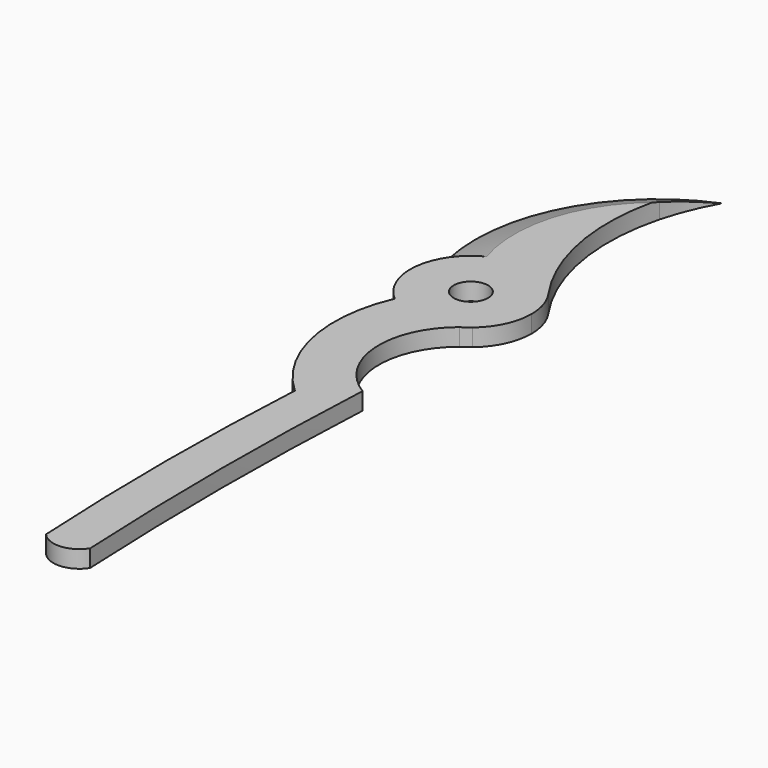
from build123d import *

# Parameters (mm, degrees)
F0_R     = 3.97
F1_DEPTH = 4
F2_SIZE2 = 3.99999
F2_SIZE  = 8.99999


# Not quite as in the source:
# - a fillet or chamfer is up to 0.001 mm smaller than in the source, because OpenCascade refuses the exact size


with BuildPart() as f1:
    # F0 (on Top) → F1 (new body)
    with BuildSketch(Plane.XY):
        with BuildLine():
            ThreePointArc((-1.9595979293, -1.3771342837), (-1.0019520075, -0.6570443939), (0, 0))
            Line((0, 0), (-18, 0))
            ThreePointArc((-18, 0), (-10.1975519696, -3.2248817144), (-1.9595979293, -1.3771342837))
        make_face()
        with BuildLine():
            Line((-18, 0), (0, 0))
            ThreePointArc((0, 0), (3.6885775404, 4.8077255117), (5, 10.7238052948))
            ThreePointArc((5, 10.7238052948), (4.3572555803, 14.9171003433), (2.4880395194, 18.7253643928))
            ThreePointArc((2.4880395194, 18.7253643928), (-5.3400778901, 24.2369459419), (-14.8797121879, 23.4292759507))
            ThreePointArc((-14.8797121879, 23.4292759507), (-19.2476875403, 20.262405825), (-22.0937623429, 15.6789428013))
            ThreePointArc((-22.0937623429, 15.6789428013), (-22.5458811252, 7.1869840464), (-18, 0))
        make_face()
        with Locations((-9, 10.7238052948)):
            Circle(F0_R, mode=Mode.SUBTRACT)
        with BuildLine():
            ThreePointArc((-1.9595979293, -1.3771342837), (-0.9502950764, -0.7305498003), (0, 0))
            ThreePointArc((0, 0), (-1.0019520075, -0.6570443939), (-1.9595979293, -1.3771342837))
        make_face()
        with BuildLine():
            ThreePointArc((-1.9595979293, -1.3771342837), (-10.1975519696, -3.2248817144), (-18, 0))
            ThreePointArc((-18, 0), (-20.1233033288, -20.9955621955), (-9.6223697705, -39.3))
            ThreePointArc((-9.6223697705, -39.3), (-10.6300458729, -75.2), (-9.6223697705, -111.1))
            ThreePointArc((-9.6223697705, -111.1), (-4.6347237623, -113.1756773925), (0, -110.4))
            ThreePointArc((0, -110.4), (-1.0035695792, -71.1), (0, -31.8))
            ThreePointArc((0, -31.8), (-8.8818164322, -17.0975519696), (-1.9595979293, -1.3771342837))
        make_face()
        with BuildLine():
            ThreePointArc((0, 71.9253643928), (-22.9860499931, 48.4918947584), (-22.0937623429, 15.6789428013))
            ThreePointArc((-22.0937623429, 15.6789428013), (-19.2476875403, 20.262405825), (-14.8797121879, 23.4292759507))
            ThreePointArc((-14.8797121879, 23.4292759507), (-15.2779476248, 43.1630862457), (-4.8626121432, 59.9292022847))
            ThreePointArc((-4.8626121432, 59.9292022847), (-2.821148436, 66.0853048958), (0, 71.9253643928))
        make_face()
        with BuildLine():
            ThreePointArc((-14.8797121879, 23.4292759507), (-5.3400778901, 24.2369459419), (2.4880395194, 18.7253643928))
            ThreePointArc((2.4880395194, 18.7253643928), (-5.7061096076, 38.5211376574), (-4.8626121432, 59.9292022847))
            ThreePointArc((-4.8626121432, 59.9292022847), (-15.2779476248, 43.1630862457), (-14.8797121879, 23.4292759507))
        make_face()
    extrude(amount=F1_DEPTH)

    # F2 (size 9 and 4 in the source; OpenCascade refuses exactly that, so slightly less here)
    f2_edges = [f1.edges().sort_by_distance(p)[0] for p in [
        (-22.98605, 48.491895, 4),
    ]]
    f2_side = f1.faces().sort_by_distance((-10.106545, -9.722551, 4))[0]
    chamfer(f2_edges, length=F2_SIZE, length2=F2_SIZE2, reference=f2_side)


solid = f1.part
